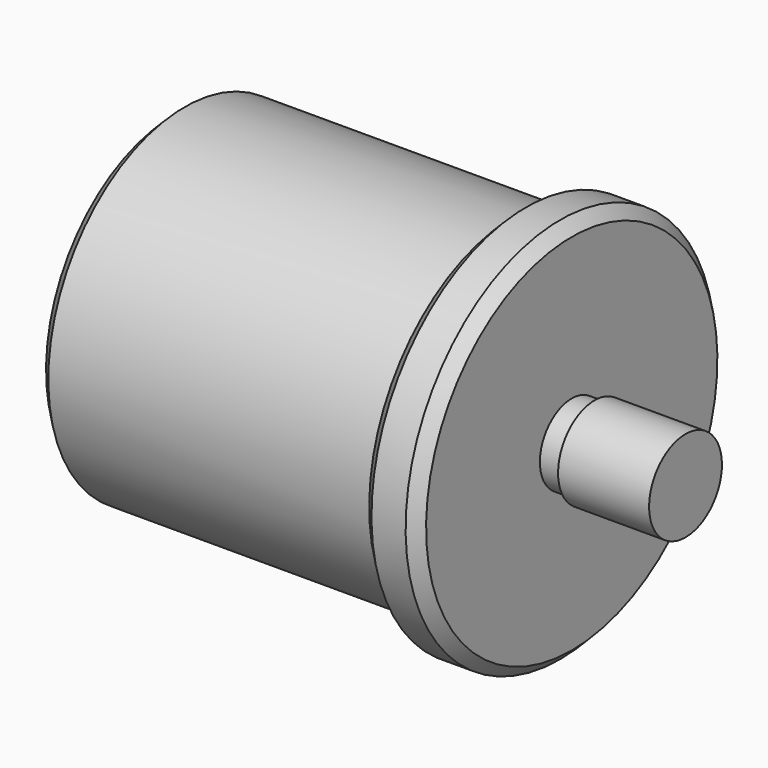
from build123d import *

# Parameters (mm, degrees)
F2_SIZE = 1


with BuildPart() as f1:
    # F0 (on Front) → F1 (revolve)
    with BuildSketch(Plane.XZ):
        Polygon((-72.3989970755, 34.4926873816), (-72.3989970755, 19.4926873816), (-42.3989970755, 19.4926873816), (-42.3989970755, 17.4926873816), (-37.3989970755, 17.4926873816), (-37.3989970755, 30.4926873816), (-37.3989970755, 30.9926873816), (-35.3989970755, 30.9926873816), (-35.3989970755, 30.4926873816), (-27.3989970755, 30.4926873816), (-27.3989970755, 34.4926873816), align=None)
    revolve(axis=Axis((-49.8989970755, 0, 34.4926873816), (-1, 0, 0)))

    # F2
    f2_edges = [f1.edges().sort_by_distance(p)[0] for p in [
        (-37.398997, 0, 51.492687),
        (-42.398997, 0, 51.492687),
        (-72.398997, 0, 49.492687),
    ]]
    chamfer(f2_edges, length=F2_SIZE)


solid = f1.part
